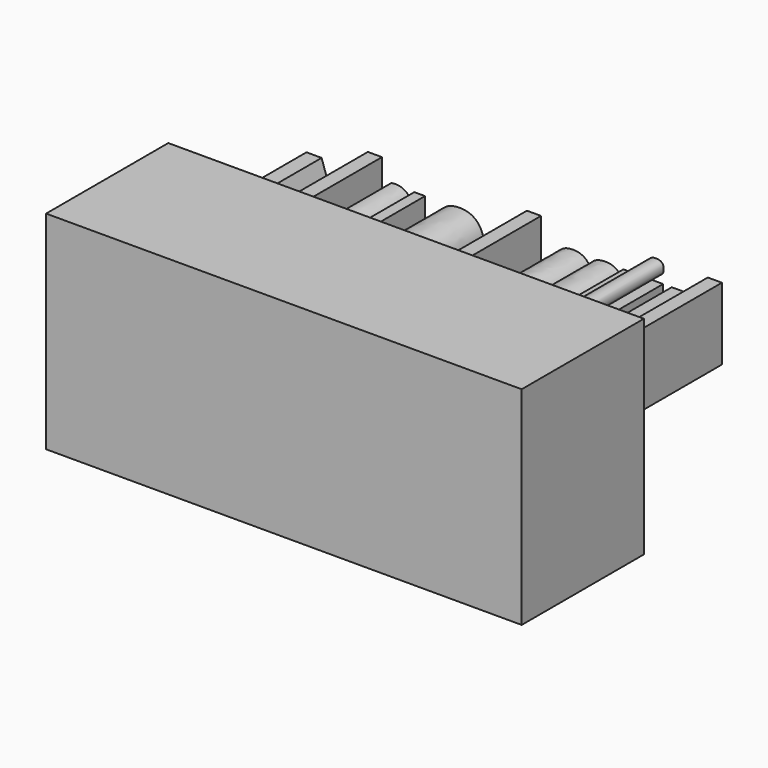
from build123d import *

# Parameters (mm, degrees)
F0_W         = 79.0938585997
F0_H         = 34.5081314445
F1_DEPTH     = 25.4
F2_TEXT_SIZE = 15.770713655
F3_DEPTH     = 25.4


# Not quite as in the source:
# - Text() gives the source's letters only with a copy of the font that has no kerning and outlines rounded to 1/6400 em; it was checked with that copy


with BuildPart() as f1:
    # F0 (on Front) → F1 (new body)
    with BuildSketch(Plane.XZ):
        with Locations((3.0538141727, 26.873588562)):
            Rectangle(F0_W, F0_H)
    extrude(amount=F1_DEPTH)

    # F2 (on face) → F3 (join)
    with BuildSketch(Plane(origin=(0, 0, 0), x_dir=(-1, 0, 0), z_dir=(0, 1, 0))):
        with Locations((-36.4931151271, 24.7066413156)):
            Text('kimberly', F2_TEXT_SIZE, font='Open Sans', font_style=FontStyle.BOLD, text_align=(TextAlign.LEFT, TextAlign.BOTTOM))
    extrude(amount=F3_DEPTH)


solid = f1.part
